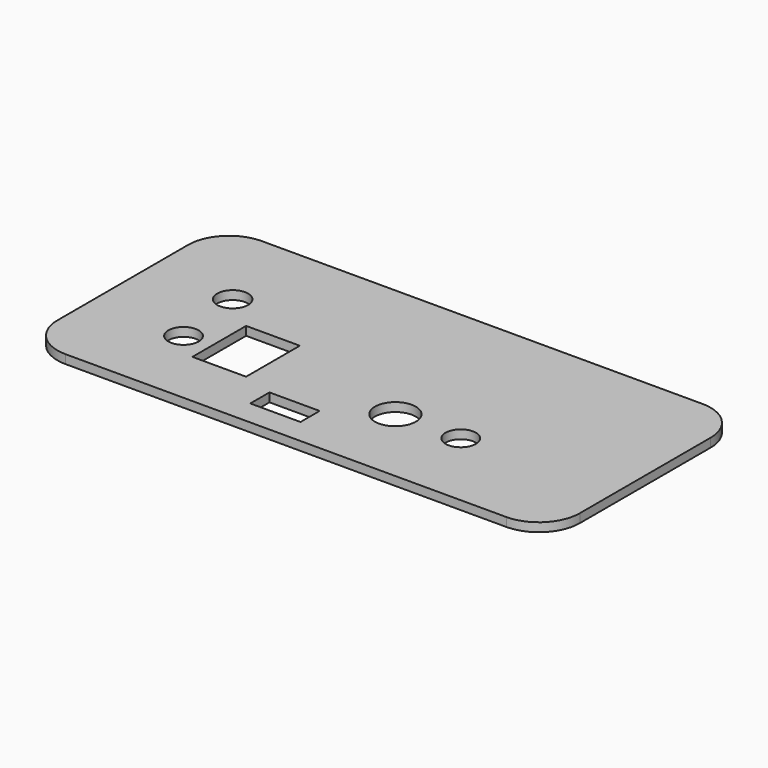
from build123d import *

# Parameters (mm, degrees)
F0_W     = 8.6
F0_H     = 4.1
F0_W_2   = 9.2
F0_H_2   = 11.5
F1_DEPTH = 1.5
F2_D     = 5.2
F2_DEPTH = 2
F2_TIP   = 1.5622376095
F3_D     = 7
F3_DEPTH = 2
F3_TIP   = 2.1030121666
F4_D     = 5.3
F4_DEPTH = 2
F4_TIP   = 1.5922806404


# Not quite as in the source:
# - a feature names something its author has since deleted; it is built from what else it names


with BuildPart() as f1:
    # F0 (on Top) → F1 (new body)
    with BuildSketch(Plane.XY):
        with BuildLine():
            Line((-37.75, -21), (37.75, -21))
            ThreePointArc((37.75, -21), (42.6997474683, -18.9497474683), (44.75, -14))
            Line((44.75, -14), (44.75, 14))
            ThreePointArc((44.75, 14), (42.6997474683, 18.9497474683), (37.75, 21))
            Line((37.75, 21), (-37.75, 21))
            ThreePointArc((-37.75, 21), (-42.6997474683, 18.9497474683), (-44.75, 14))
            Line((-44.75, 14), (-44.75, -14))
            ThreePointArc((-44.75, -14), (-42.6997474683, -18.9497474683), (-37.75, -21))
        make_face()
        with Locations((-5.25, -14.65)):
            Rectangle(F0_W, F0_H, mode=Mode.SUBTRACT)
        with Locations((-19.43, -5.25)):
            Rectangle(F0_W_2, F0_H_2, mode=Mode.SUBTRACT)
    extrude(amount=F1_DEPTH)

    # F2
    with Locations(Plane(origin=(0, 0, 0), x_dir=(1, 0, 0), z_dir=(0, 0, -1))):
        with Locations((18.75, 7), (-28.75, 7)):
            Hole(F2_D / 2, depth=F2_DEPTH)
            with Locations((0, 0, -(F2_DEPTH + F2_TIP / 2))):  # 118° drill point
                Cone(0, F2_D / 2, F2_TIP, mode=Mode.SUBTRACT)

    # F3
    with Locations(Plane(origin=(0, 0, 0), x_dir=(1, 0, 0), z_dir=(0, 0, -1))):
        with Locations((7.55, 7)):
            Hole(F3_D / 2, depth=F3_DEPTH)
            with Locations((0, 0, -(F3_DEPTH + F3_TIP / 2))):  # 118° drill point
                Cone(0, F3_D / 2, F3_TIP, mode=Mode.SUBTRACT)

    # F4
    with Locations(Plane(origin=(0, 0, 0), x_dir=(1, 0, 0), z_dir=(0, 0, -1))):
        with Locations((-30.2482247353, -5.4)):
            Hole(F4_D / 2, depth=F4_DEPTH)
            with Locations((0, 0, -(F4_DEPTH + F4_TIP / 2))):  # 118° drill point
                Cone(0, F4_D / 2, F4_TIP, mode=Mode.SUBTRACT)


solid = f1.part
